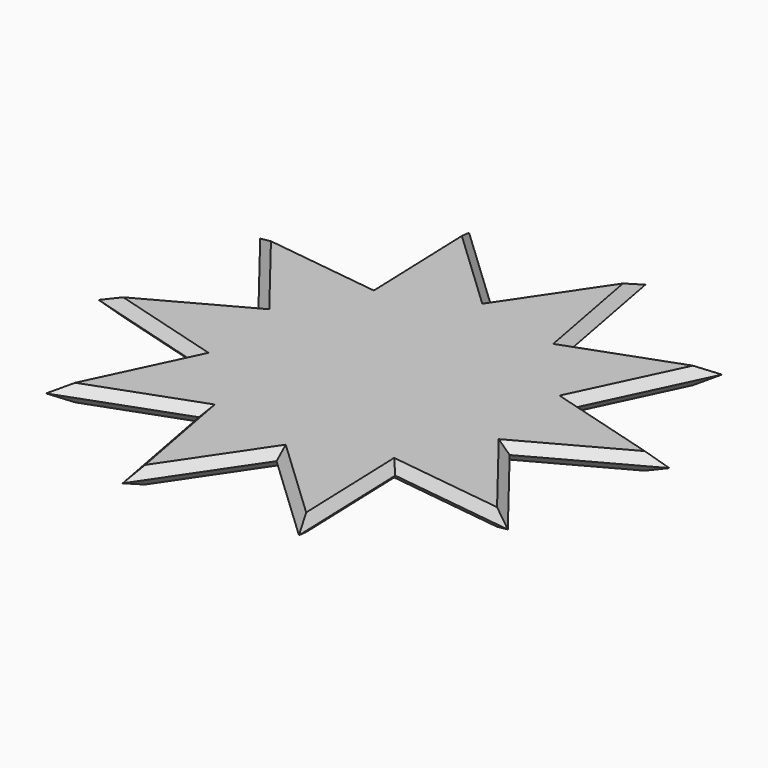
from build123d import *

# Parameters (mm, degrees)
F1_DEPTH = 3.175
F2_SIZE  = 3.17499


# Not quite as in the source:
# - a fillet or chamfer is up to 0.001 mm smaller than in the source, because OpenCascade refuses the exact size


with BuildPart() as f1:
    # F0 (on Top) → F1 (new body, symmetric)
    with BuildSketch(Plane.XY):
        with BuildLine():
            Line((28.5780178367, 49.3127499276), (9.3443886308, 42.3114214845))
            Line((9.3443886308, 42.3114214845), (19.4354125913, 32.7700280349))
            ThreePointArc((19.4354125913, 32.7700280349), (19.9071953157, 32.4855902619), (20.374816102, 32.1943608231))
            Line((20.374816102, 32.1943608231), (32.4297987565, 28.7381652083))
            Line((32.4297987565, 28.7381652083), (28.5780178367, 49.3127499276))
        make_face()
        Polygon((17.3102603478, -39.723152866), (5.865205062, -56.692590155), (39.6851250968, -88.6704315269), (38.068118978, -42.4177878534), align=None)
        with BuildLine():
            Line((55.7303053322, -11.9408323194), (43.1281280055, 4.1879065968))
            Line((43.1281280055, 4.1879065968), (37.1720214851, -8.3576802229))
            ThreePointArc((37.1720214851, -8.3576802229), (37.0472939672, -8.8942683629), (36.9148210816, -9.4289970047))
            Line((36.9148210816, -9.4289970047), (37.3529782276, -21.961989993))
            Line((37.3529782276, -21.961989993), (55.7303053322, -11.9408323194))
        make_face()
        Polygon((-39.6851250968, 88.6704315269), (-38.068118978, 42.4177878534), (-17.3102603478, 39.723152866), (-5.865205062, 56.692590155), align=None)
        with BuildLine():
            Line((52.1054092529, 23.0971153067), (32.4297987565, 28.7381652083))
            Line((32.4297987565, 28.7381652083), (34.9853182751, 15.087660693))
            ThreePointArc((34.9853182751, 15.087660693), (35.1998101887, 14.5802387731), (35.4069429826, 14.069768606))
            Line((35.4069429826, 14.069768606), (43.1281280055, 4.1879065968))
            Line((43.1281280055, 4.1879065968), (52.1054092529, 23.0971153067))
        make_face()
        Polygon((37.3529782276, -21.961989993), (38.068118978, -42.4177878534), (84.2251125931, -48.4095547365), (55.7303053322, -11.9408323194), align=None)
        with BuildLine():
            ThreePointArc((25.1602759184, -28.6106713607), (24.7439706414, -28.9714672894), (24.322492216, -29.3262062395))
            Line((24.322492216, -29.3262062395), (17.3102603478, -39.723152866))
            Line((17.3102603478, -39.723152866), (38.068118978, -42.4177878534))
            Line((38.068118978, -42.4177878534), (37.3529782276, -21.961989993))
            Line((37.3529782276, -21.961989993), (25.1602759184, -28.6106713607))
        make_face()
        Polygon((-55.7303053322, 11.9408323194), (-37.3529782276, 21.961989993), (-38.068118978, 42.4177878534), (-84.2251125931, 48.4095547365), align=None)
        Polygon((96.5939697852, 10.342126583), (52.1054092529, 23.0971153067), (43.1281280055, 4.1879065968), (55.7303053322, -11.9408323194), align=None)
        with BuildLine():
            ThreePointArc((3.5381601171, -37.9353584797), (2.9892915472, -37.9825504152), (2.4397980151, -38.0218014519))
            Line((2.4397980151, -38.0218014519), (-9.3443886308, -42.3114214845))
            Line((-9.3443886308, -42.3114214845), (5.865205062, -56.692590155))
            Line((5.865205062, -56.692590155), (17.3102603478, -39.723152866))
            Line((17.3102603478, -39.723152866), (3.5381601171, -37.9353584797))
        make_face()
        Polygon((20.0132313387, 95.0622172711), (-5.865205062, 56.692590155), (9.3443886308, 42.3114214845), (28.5780178367, 49.3127499276), align=None)
        with BuildLine():
            Line((-38.068118978, 42.4177878534), (-37.3529782276, 21.961989993))
            Line((-37.3529782276, 21.961989993), (-25.1602759184, 28.6106713607))
            ThreePointArc((-25.1602759184, 28.6106713607), (-24.7439706414, 28.9714672894), (-24.322492216, 29.3262062395))
            Line((-24.322492216, 29.3262062395), (-17.3102603478, 39.723152866))
            Line((-17.3102603478, 39.723152866), (-38.068118978, 42.4177878534))
        make_face()
        Polygon((72.0672136275, 65.1434670637), (28.5780178367, 49.3127499276), (32.4297987565, 28.7381652083), (52.1054092529, 23.0971153067), align=None)
        with BuildLine():
            ThreePointArc((-19.4354125913, -32.7700280349), (-19.9071953157, -32.4855902619), (-20.374816102, -32.1943608231))
            Line((-20.374816102, -32.1943608231), (-32.4297987565, -28.7381652083))
            Line((-32.4297987565, -28.7381652083), (-28.5780178367, -49.3127499276))
            Line((-28.5780178367, -49.3127499276), (-9.3443886308, -42.3114214845))
            Line((-9.3443886308, -42.3114214845), (-19.4354125913, -32.7700280349))
        make_face()
        Polygon((-52.1054092529, -23.0971153067), (-43.1281280055, -4.1879065968), (-55.7303053322, 11.9408323194), (-96.5939697852, -10.342126583), align=None)
        with BuildLine():
            ThreePointArc((-34.9853182751, -15.087660693), (-35.1998101887, -14.5802387731), (-35.4069429826, -14.069768606))
            Line((-35.4069429826, -14.069768606), (-43.1281280055, -4.1879065968))
            Line((-43.1281280055, -4.1879065968), (-52.1054092529, -23.0971153067))
            Line((-52.1054092529, -23.0971153067), (-32.4297987565, -28.7381652083))
            Line((-32.4297987565, -28.7381652083), (-34.9853182751, -15.087660693))
        make_face()
        Polygon((-32.4297987565, -28.7381652083), (-52.1054092529, -23.0971153067), (-72.0672136275, -65.1434670637), (-28.5780178367, -49.3127499276), align=None)
        with BuildLine():
            ThreePointArc((-37.1720214851, 8.3576802229), (-37.0472939672, 8.8942683629), (-36.9148210816, 9.4289970047))
            Line((-36.9148210816, 9.4289970047), (-37.3529782276, 21.961989993))
            Line((-37.3529782276, 21.961989993), (-55.7303053322, 11.9408323194))
            Line((-55.7303053322, 11.9408323194), (-43.1281280055, -4.1879065968))
            Line((-43.1281280055, -4.1879065968), (-37.1720214851, 8.3576802229))
        make_face()
        Polygon((-9.3443886308, -42.3114214845), (-28.5780178367, -49.3127499276), (-20.0132313387, -95.0622172711), (5.865205062, -56.692590155), align=None)
        with BuildLine():
            Line((-5.865205062, 56.692590155), (-17.3102603478, 39.723152866))
            Line((-17.3102603478, 39.723152866), (-3.5381601171, 37.9353584797))
            ThreePointArc((-3.5381601171, 37.9353584797), (-2.9892915472, 37.9825504152), (-2.4397980151, 38.0218014519))
            Line((-2.4397980151, 38.0218014519), (9.3443886308, 42.3114214845))
            Line((9.3443886308, 42.3114214845), (-5.865205062, 56.692590155))
        make_face()
        with BuildLine():
            ThreePointArc((-25.1602759184, 28.6106713607), (-32.4855902619, 19.9071953157), (-36.9148210816, 9.4289970047))
            ThreePointArc((-36.9148210816, 9.4289970047), (-37.0472939672, 8.8942683629), (-37.1720214851, 8.3576802229))
            ThreePointArc((-37.1720214851, 8.3576802229), (-37.9825504152, -2.9892915472), (-35.4069429826, -14.069768606))
            ThreePointArc((-35.4069429826, -14.069768606), (-35.1998101887, -14.5802387731), (-34.9853182751, -15.087660693))
            ThreePointArc((-34.9853182751, -15.087660693), (-28.9714672894, -24.7439706414), (-20.374816102, -32.1943608231))
            ThreePointArc((-20.374816102, -32.1943608231), (-19.9071953157, -32.4855902619), (-19.4354125913, -32.7700280349))
            ThreePointArc((-19.4354125913, -32.7700280349), (-8.8942683629, -37.0472939672), (2.4397980151, -38.0218014519))
            ThreePointArc((2.4397980151, -38.0218014519), (2.9892915472, -37.9825504152), (3.5381601171, -37.9353584797))
            ThreePointArc((3.5381601171, -37.9353584797), (14.5802387731, -35.1998101887), (24.322492216, -29.3262062395))
            ThreePointArc((24.322492216, -29.3262062395), (24.7439706414, -28.9714672894), (25.1602759184, -28.6106713607))
            ThreePointArc((25.1602759184, -28.6106713607), (32.4855902619, -19.9071953157), (36.9148210816, -9.4289970047))
            ThreePointArc((36.9148210816, -9.4289970047), (37.0472939672, -8.8942683629), (37.1720214851, -8.3576802229))
            ThreePointArc((37.1720214851, -8.3576802229), (37.9825504152, 2.9892915472), (35.4069429826, 14.069768606))
            ThreePointArc((35.4069429826, 14.069768606), (35.1998101887, 14.5802387731), (34.9853182751, 15.087660693))
            ThreePointArc((34.9853182751, 15.087660693), (28.9714672894, 24.7439706414), (20.374816102, 32.1943608231))
            ThreePointArc((20.374816102, 32.1943608231), (19.9071953157, 32.4855902619), (19.4354125913, 32.7700280349))
            ThreePointArc((19.4354125913, 32.7700280349), (8.8942683629, 37.0472939672), (-2.4397980151, 38.0218014519))
            ThreePointArc((-2.4397980151, 38.0218014519), (-2.9892915472, 37.9825504152), (-3.5381601171, 37.9353584797))
            ThreePointArc((-3.5381601171, 37.9353584797), (-14.5802387731, 35.1998101887), (-24.322492216, 29.3262062395))
            ThreePointArc((-24.322492216, 29.3262062395), (-24.7439706414, 28.9714672894), (-25.1602759184, 28.6106713607))
        make_face()
        with BuildLine():
            ThreePointArc((-20.374816102, -32.1943608231), (-28.9714672894, -24.7439706414), (-34.9853182751, -15.087660693))
            Line((-34.9853182751, -15.087660693), (-32.4297987565, -28.7381652083))
            Line((-32.4297987565, -28.7381652083), (-20.374816102, -32.1943608231))
        make_face()
        with BuildLine():
            ThreePointArc((2.4397980151, -38.0218014519), (-8.8942683629, -37.0472939672), (-19.4354125913, -32.7700280349))
            Line((-19.4354125913, -32.7700280349), (-9.3443886308, -42.3114214845))
            Line((-9.3443886308, -42.3114214845), (2.4397980151, -38.0218014519))
        make_face()
        with BuildLine():
            ThreePointArc((24.322492216, -29.3262062395), (14.5802387731, -35.1998101887), (3.5381601171, -37.9353584797))
            Line((3.5381601171, -37.9353584797), (17.3102603478, -39.723152866))
            Line((17.3102603478, -39.723152866), (24.322492216, -29.3262062395))
        make_face()
        with BuildLine():
            ThreePointArc((36.9148210816, -9.4289970047), (32.4855902619, -19.9071953157), (25.1602759184, -28.6106713607))
            Line((25.1602759184, -28.6106713607), (37.3529782276, -21.961989993))
            Line((37.3529782276, -21.961989993), (36.9148210816, -9.4289970047))
        make_face()
        with BuildLine():
            Line((43.1281280055, 4.1879065968), (35.4069429826, 14.069768606))
            ThreePointArc((35.4069429826, 14.069768606), (37.9825504152, 2.9892915472), (37.1720214851, -8.3576802229))
            Line((37.1720214851, -8.3576802229), (43.1281280055, 4.1879065968))
        make_face()
        with BuildLine():
            Line((32.4297987565, 28.7381652083), (20.374816102, 32.1943608231))
            ThreePointArc((20.374816102, 32.1943608231), (28.9714672894, 24.7439706414), (34.9853182751, 15.087660693))
            Line((34.9853182751, 15.087660693), (32.4297987565, 28.7381652083))
        make_face()
        with BuildLine():
            Line((9.3443886308, 42.3114214845), (-2.4397980151, 38.0218014519))
            ThreePointArc((-2.4397980151, 38.0218014519), (8.8942683629, 37.0472939672), (19.4354125913, 32.7700280349))
            Line((19.4354125913, 32.7700280349), (9.3443886308, 42.3114214845))
        make_face()
        with BuildLine():
            Line((-17.3102603478, 39.723152866), (-24.322492216, 29.3262062395))
            ThreePointArc((-24.322492216, 29.3262062395), (-14.5802387731, 35.1998101887), (-3.5381601171, 37.9353584797))
            Line((-3.5381601171, 37.9353584797), (-17.3102603478, 39.723152866))
        make_face()
        with BuildLine():
            ThreePointArc((-35.4069429826, -14.069768606), (-37.9825504152, -2.9892915472), (-37.1720214851, 8.3576802229))
            Line((-37.1720214851, 8.3576802229), (-43.1281280055, -4.1879065968))
            Line((-43.1281280055, -4.1879065968), (-35.4069429826, -14.069768606))
        make_face()
        with BuildLine():
            Line((-37.3529782276, 21.961989993), (-36.9148210816, 9.4289970047))
            ThreePointArc((-36.9148210816, 9.4289970047), (-32.4855902619, 19.9071953157), (-25.1602759184, 28.6106713607))
            Line((-25.1602759184, 28.6106713607), (-37.3529782276, 21.961989993))
        make_face()
    extrude(amount=F1_DEPTH, both=True)

    # F2 (size 3.175 in the source; OpenCascade refuses exactly that, so slightly less here)
    f2_edges = [f1.edges().sort_by_distance(p)[0] for p in [
        (22.775165, -72.681511, 3.175),
        (38.876622, -65.54411, 3.175),
        (61.146616, -45.413671, 3.175),
        (69.977709, -30.175194, 3.175),
        (76.162138, -0.799353, 3.175),
        (74.34969, 16.719621, 3.175),
        (62.086311, 44.120291, 3.175),
        (50.322616, 57.228108, 3.175),
        (24.295625, 72.187484, 3.175),
        (7.074013, 75.877404, 3.175),
        (-22.775165, 72.681511, 3.175),
        (-38.876622, 65.54411, 3.175),
        (-61.146616, 45.413671, 3.175),
        (-69.977709, 30.175194, 3.175),
        (-76.162138, 0.799353, 3.175),
        (-74.34969, -16.719621, 3.175),
        (-62.086311, -44.120291, 3.175),
        (-50.322616, -57.228108, 3.175),
        (-24.295625, -72.187484, 3.175),
        (-7.074013, -75.877404, 3.175),
        (22.775165, -72.681511, -3.175),
        (38.876622, -65.54411, -3.175),
        (61.146616, -45.413671, -3.175),
        (69.977709, -30.175194, -3.175),
        (76.162138, -0.799353, -3.175),
        (74.34969, 16.719621, -3.175),
        (62.086311, 44.120291, -3.175),
        (50.322616, 57.228108, -3.175),
        (24.295625, 72.187484, -3.175),
        (7.074013, 75.877404, -3.175),
        (-22.775165, 72.681511, -3.175),
        (-38.876622, 65.54411, -3.175),
        (-61.146616, 45.413671, -3.175),
        (-69.977709, 30.175194, -3.175),
        (-76.162138, 0.799353, -3.175),
        (-74.34969, -16.719621, -3.175),
        (-62.086311, -44.120291, -3.175),
        (-50.322616, -57.228108, -3.175),
        (-24.295625, -72.187484, -3.175),
        (-7.074013, -75.877404, -3.175),
    ]]
    chamfer(f2_edges, length=F2_SIZE)


solid = f1.part
